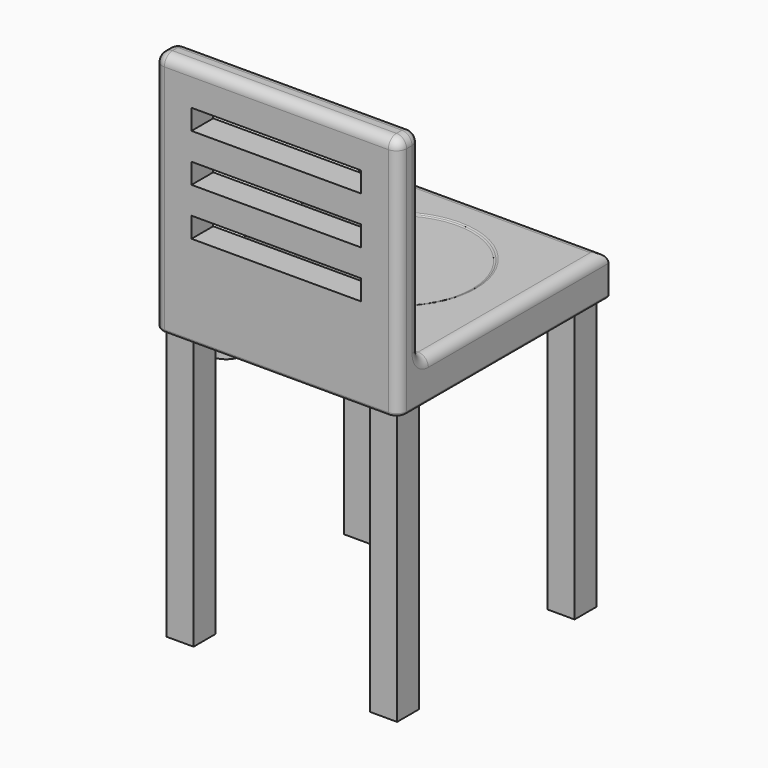
from build123d import *

# Parameters (mm, degrees)
F2_W      = 457.2
F2_H      = 457.2
F3_DEPTH  = 50.8
F0_W      = 457.2
F0_H      = 457.2
F4_DEPTH  = 76.2
F5_W      = 50.8
F5_H      = 50.8
F6_DEPTH  = 508
F7_R      = 19.05
F8_W      = 317.5
F8_H      = 38.1
F9_DEPTH  = 63.5
F10_R     = 31.7295136587
F10_R_2   = 22.617106641
F11_DEPTH = 63.5
F12_R     = 147.0598184699
F13_DEPTH = 2.54
F15_R     = 5.08
F16_R     = 5.08


# Not quite as in the source:
# - a fillet or chamfer that OpenCascade refuses, or shapes differently, is made with other operations: its cross-section is extruded or revolved along the edge and cut away or added


with BuildPart() as f3:
    # F2 (on offset) → F3 (new body)
    with BuildSketch(Plane.XZ.offset(228.6)):
        with Locations((-0.6349999458, 228.6)):
            Rectangle(F2_W, F2_H)
    extrude(amount=F3_DEPTH)

    # F0 (on Top) → F4 (join)
    with BuildSketch(Plane.XY):
        with Locations((-0.6349999458, -16.5623649633)):
            Rectangle(F0_W, F0_H)
    extrude(amount=F4_DEPTH)

    # F5 (on face) → F6 (join)
    with BuildSketch(Plane(origin=(0, 0, 0), x_dir=(1, 0, 0), z_dir=(0, 0, -1))):
        with Locations((-191.1349999458, 241.3)):
            Rectangle(F5_W, F5_H)
        with Locations((189.8650000542, 241.3)):
            Rectangle(F5_W, F5_H)
        with Locations((189.8650000542, -173.9376350367)):
            Rectangle(F5_W, F5_H)
        with Locations((-191.1349999458, -173.9376350367)):
            Rectangle(F5_W, F5_H)
    extrude(amount=F6_DEPTH)

    # F7
    f7_edges = [f3.edges().sort_by_distance(p)[0] for p in [
        (-0.635, -228.6, 76.2),
        (-0.635, -228.6, 457.2),
        (-229.235, -228.6, 266.7),
        (227.965, -228.6, 266.7),
        (-0.635, -279.4, 457.2),
        (227.965, -279.4, 228.6),
        (227.965, -254, 457.2),
        (-229.235, -254, 457.2),
        (-229.235, -8.281182, 76.2),
        (227.965, -8.281182, 76.2),
        (-0.635, 212.037635, 76.2),
        (-229.235, -279.4, 228.6),
    ]]
    fillet(f7_edges, radius=F7_R)

    # F8 (on face) → F9 (cut, symmetric)
    with BuildSketch(Plane.XZ.offset(279.4)):
        with Locations((-0.6349999458, 368.3)):
            Rectangle(F8_W, F8_H)
        with Locations((-0.6349999458, 279.4)):
            Rectangle(F8_W, F8_H)
        with Locations((-0.6349999458, 190.5)):
            Rectangle(F8_W, F8_H)
    extrude(amount=F9_DEPTH, both=True, mode=Mode.SUBTRACT)

    # F10 (on face) → F11 (join)
    with BuildSketch(Plane(origin=(0, 0, 0), x_dir=(1, 0, 0), z_dir=(0, 0, -1))):
        with Locations((-183.2177340984, 168.4852540493)):
            Circle(F10_R)
        with Locations((-183.2177340984, 168.4852540493)):
            Circle(F10_R_2, mode=Mode.SUBTRACT)
    extrude(amount=F11_DEPTH)

    # F12 (on face) → F13 (cut)
    with BuildSketch(Plane.XY.offset(76.2)):
        Circle(F12_R)
    extrude(amount=-F13_DEPTH, mode=Mode.SUBTRACT)

    # F14: fillet of radius 5.08 on 1 edges, made by hand

    # F14_s1 → F14_t2 (revolve)
    with BuildSketch(Plane.XZ):
        with BuildLine():
            ThreePointArc((147.0598184699, 76.2), (145.2004094187, 74.3405909488), (142.6604094187, 73.66))
            Line((142.6604094187, 73.66), (147.0598184699, 73.66))
            Line((147.0598184699, 73.66), (147.0598184699, 76.2))
        make_face()
    revolve(axis=Axis((0, 0, 73.66), (0, 0, 1)))

    # F15
    f15_edges = [f3.edges().sort_by_distance(p)[0] for p in [
        (-147.059818, 0, 76.2),
    ]]
    fillet(f15_edges, radius=F15_R)

    # F16
    f16_edges = [f3.edges().sort_by_distance(p)[0] for p in [
        (-229.235, -24.156182, 0),
        (-0.635, 212.037635, 0),
        (227.965, -24.156182, 0),
        (-0.635, -279.4, 0),
        (222.385384, -273.820384, 0),
        (-223.655384, -273.820384, 0),
    ]]
    fillet(f16_edges, radius=F16_R)


solid = f3.part
